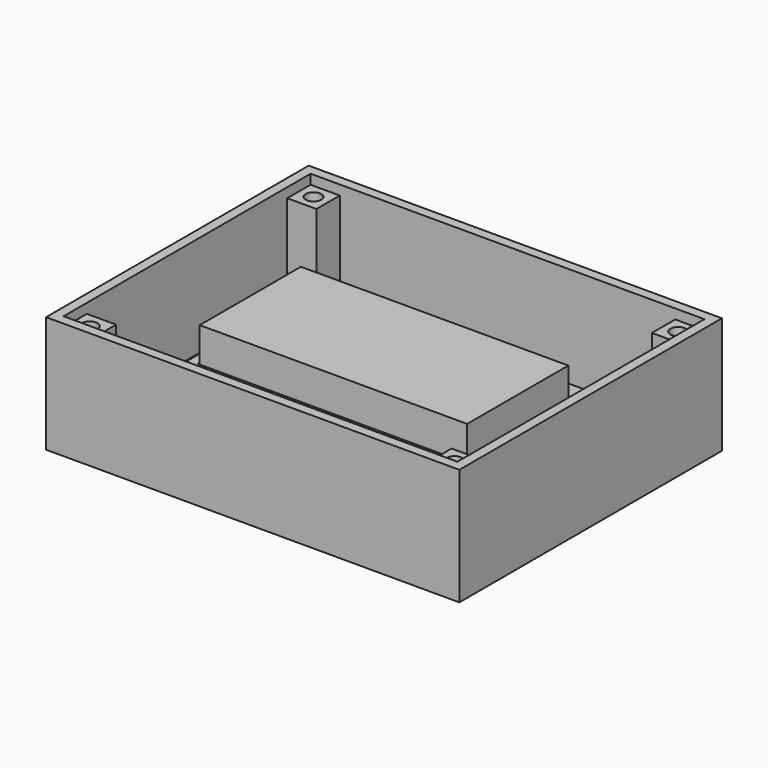
from build123d import *

# Parameters (mm, degrees)
F1_W      = 80
F1_H      = 62.5
F1_R      = 1.5
F2_DEPTH  = 1.6
F3_W      = 85
F3_H      = 67.5
F3_W_2    = 6
F3_H_2    = 6
F3_R      = 1.6
F4_DEPTH  = 2
F5_DEPTH  = 22
F6_W      = 6
F6_H      = 6
F6_R      = 1.6
F7_DEPTH  = 2
F8_W      = 55
F8_H      = 26
F9_DEPTH  = 17
F10_W     = 59.4
F10_H     = 30.4
F10_W_2   = 55.4
F10_H_2   = 26.4
F11_DEPTH = 10


with BuildPart() as f2:
    # F1 (on Top) → F2 (new body)
    with BuildSketch(Plane.XY):
        Rectangle(F1_W, F1_H)
        with Locations((-37.5, -28.75)):
            Circle(F1_R, mode=Mode.SUBTRACT)
        with Locations((-37.5, -2.25)):
            Circle(F1_R, mode=Mode.SUBTRACT)
        with Locations((37.5, -28.75)):
            Circle(F1_R, mode=Mode.SUBTRACT)
        with Locations((37.5, -2.25)):
            Circle(F1_R, mode=Mode.SUBTRACT)
        with Locations((-37.5, 28.75)):
            Circle(F1_R, mode=Mode.SUBTRACT)
        with Locations((37.5, 28.75)):
            Circle(F1_R, mode=Mode.SUBTRACT)
    extrude(amount=F2_DEPTH)


with BuildPart() as f4:
    # F3 (on Top) → F4 (new body)
    with BuildSketch(Plane.XY):
        Rectangle(F3_W, F3_H)
        Polygon((34.5, 31.75), (40.5, 31.75), (40.5, 25.75), (40.5, -25.75), (40.5, -31.75), (34.5, -31.75), (-34.5, -31.75), (-40.5, -31.75), (-40.5, -25.75), (-40.5, 25.75), (-40.5, 31.75), (-34.5, 31.75), align=None, mode=Mode.SUBTRACT)
        with Locations((-37.5, 28.75)):
            Rectangle(F3_W_2, F3_H_2)
        with Locations((-37.5, 28.75)):
            Circle(F3_R, mode=Mode.SUBTRACT)
        with Locations((-37.5, 28.75)):
            Circle(F3_R)
        Polygon((34.5, 25.75), (34.5, 31.75), (-34.5, 31.75), (-34.5, 25.75), (-40.5, 25.75), (-40.5, -25.75), (-34.5, -25.75), (-34.5, -31.75), (34.5, -31.75), (34.5, -25.75), (40.5, -25.75), (40.5, 25.75), align=None)
        with Locations((37.5, 28.75)):
            Rectangle(F3_W_2, F3_H_2)
        with Locations((37.5, 28.75)):
            Circle(F3_R, mode=Mode.SUBTRACT)
        with Locations((37.5, 28.75)):
            Circle(F3_R)
        with Locations((37.5, -28.75)):
            Rectangle(F3_W_2, F3_H_2)
        with Locations((37.5, -28.75)):
            Circle(F3_R, mode=Mode.SUBTRACT)
        with Locations((37.5, -28.75)):
            Circle(F3_R)
        with Locations((-37.5, -28.75)):
            Rectangle(F3_W_2, F3_H_2)
        with Locations((-37.5, -28.75)):
            Circle(F3_R, mode=Mode.SUBTRACT)
        with Locations((-37.5, -28.75)):
            Circle(F3_R)
    extrude(amount=-F4_DEPTH)

    # F3 (on Top) → F5 (join)
    with BuildSketch(Plane.XY):
        Rectangle(F3_W, F3_H)
        Polygon((34.5, 31.75), (40.5, 31.75), (40.5, 25.75), (40.5, -25.75), (40.5, -31.75), (34.5, -31.75), (-34.5, -31.75), (-40.5, -31.75), (-40.5, -25.75), (-40.5, 25.75), (-40.5, 31.75), (-34.5, 31.75), align=None, mode=Mode.SUBTRACT)
        with Locations((-37.5, 28.75)):
            Rectangle(F3_W_2, F3_H_2)
        with Locations((-37.5, 28.75)):
            Circle(F3_R, mode=Mode.SUBTRACT)
        with Locations((37.5, 28.75)):
            Rectangle(F3_W_2, F3_H_2)
        with Locations((37.5, 28.75)):
            Circle(F3_R, mode=Mode.SUBTRACT)
        with Locations((37.5, -28.75)):
            Rectangle(F3_W_2, F3_H_2)
        with Locations((37.5, -28.75)):
            Circle(F3_R, mode=Mode.SUBTRACT)
        with Locations((-37.5, -28.75)):
            Rectangle(F3_W_2, F3_H_2)
        with Locations((-37.5, -28.75)):
            Circle(F3_R, mode=Mode.SUBTRACT)
    extrude(amount=F5_DEPTH)

    # F6 (on face) → F7 (cut)
    with BuildSketch(Plane.XY.offset(22)):
        with Locations((-37.5, 28.75)):
            Rectangle(F6_W, F6_H)
        with Locations((-37.5, 28.75)):
            Circle(F6_R, mode=Mode.SUBTRACT)
        with Locations((-37.5, -28.75)):
            Rectangle(F6_W, F6_H)
        with Locations((-37.5, -28.75)):
            Circle(F6_R, mode=Mode.SUBTRACT)
        with Locations((37.5, 28.75)):
            Rectangle(F6_W, F6_H)
        with Locations((37.5, 28.75)):
            Circle(F6_R, mode=Mode.SUBTRACT)
        with Locations((37.5, -28.75)):
            Rectangle(F6_W, F6_H)
        with Locations((37.5, -28.75)):
            Circle(F6_R, mode=Mode.SUBTRACT)
    extrude(amount=-F7_DEPTH, mode=Mode.SUBTRACT)

    # F10 (on face) → F11 (join)
    with BuildSketch(Plane.XY):
        Rectangle(F10_W, F10_H)
        Rectangle(F10_W_2, F10_H_2, mode=Mode.SUBTRACT)
    extrude(amount=F11_DEPTH)


with BuildPart() as f9:
    # F8 (on Top) → F9 (new body)
    with BuildSketch(Plane.XY):
        Rectangle(F8_W, F8_H)
    extrude(amount=F9_DEPTH)


solid = Compound([f2.part, f4.part, f9.part])
